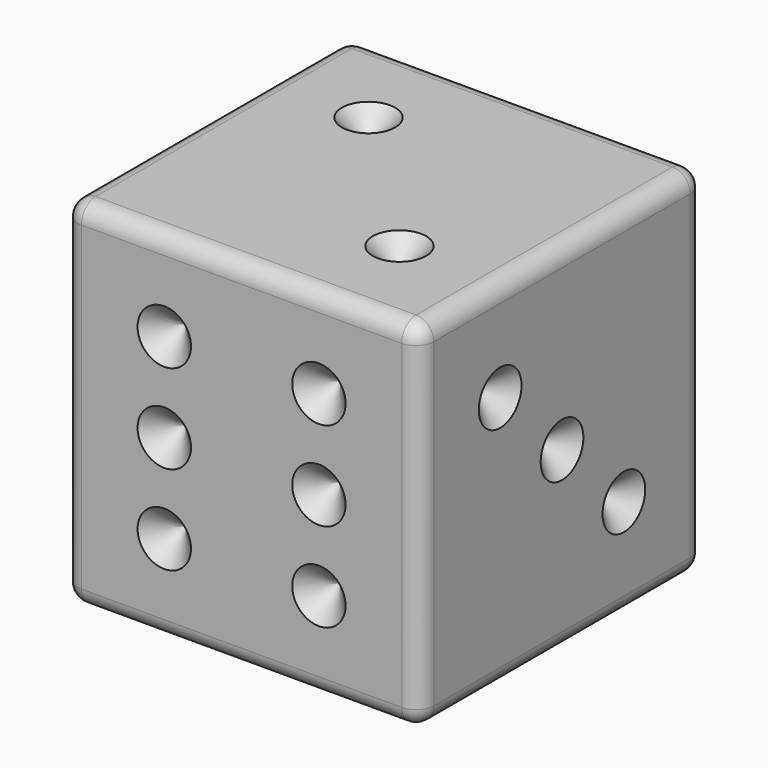
from build123d import *

# Parameters (mm, degrees)
F0_W      = 20
F0_H      = 20
F1_DEPTH  = 20
F2_R      = 1.5
F3_DEPTH  = 1.5
F4_R      = 1
F5_SIZE   = 1.49999
F6_R      = 1.5
F7_DEPTH  = 1.5
F8_SIZE   = 1.49999
F9_R      = 1.5
F10_DEPTH = 1.5
F11_SIZE  = 1.49999
F12_R     = 1.5
F13_DEPTH = 1.5
F14_SIZE  = 1.49999
F15_R     = 1.5
F16_DEPTH = 1.5
F17_SIZE  = 1.49999
F18_R     = 1.5
F19_DEPTH = 1.5
F20_SIZE  = 1.49999


# Not quite as in the source:
# - a fillet or chamfer is up to 0.001 mm smaller than in the source, because OpenCascade refuses the exact size


with BuildPart() as f1:
    # F0 (on Top) → F1 (new body)
    with BuildSketch(Plane.XY):
        with Locations((10, 10)):
            Rectangle(F0_W, F0_H)
    extrude(amount=F1_DEPTH)

    # F2 (on face) → F3 (cut)
    with BuildSketch(Plane.XY.offset(20)):
        with Locations((5.6568542495, 14.3431457505)):
            Circle(F2_R)
        with Locations((14.3431457505, 5.6568542495)):
            Circle(F2_R)
    extrude(amount=-F3_DEPTH, mode=Mode.SUBTRACT)

    # F4
    f4_edges = [f1.edges().sort_by_distance(p)[0] for p in [
        (10, 0, 20),
        (20, 0, 10),
        (0, 0, 10),
        (0, 10, 0),
        (0, 10, 20),
        (10, 20, 20),
        (20, 20, 10),
        (20, 10, 20),
        (10, 20, 0),
        (20, 10, 0),
        (0, 20, 10),
        (10, 0, 0),
    ]]
    fillet(f4_edges, radius=F4_R)

    # F5 (size 1.5 in the source; OpenCascade refuses exactly that, so slightly less here)
    f5_edges = [f1.edges().sort_by_distance(p)[0] for p in [
        (12.843146, 5.656854, 18.5),
        (4.156854, 14.343146, 18.5),
    ]]
    chamfer(f5_edges, length=F5_SIZE)

    # F6 (on face) → F7 (cut)
    with BuildSketch(Plane(origin=(0, 0, 0), x_dir=(1, 0, 0), z_dir=(0, 0, -1))):
        with Locations((5.6568542495, -5.6568542495)):
            Circle(F6_R)
        with Locations((14.3431457505, -5.6568542495)):
            Circle(F6_R)
        with Locations((14.3431457505, -14.3431457505)):
            Circle(F6_R)
        with Locations((5.6568542495, -14.3431457505)):
            Circle(F6_R)
        with Locations((10, -10)):
            Circle(F6_R)
    extrude(amount=-F7_DEPTH, mode=Mode.SUBTRACT)

    # F8 (size 1.5 in the source; OpenCascade refuses exactly that, so slightly less here)
    f8_edges = [f1.edges().sort_by_distance(p)[0] for p in [
        (4.156854, 5.656854, 1.5),
        (12.843146, 5.656854, 1.5),
        (8.5, 10, 1.5),
        (12.843146, 14.343146, 1.5),
        (4.156854, 14.343146, 1.5),
    ]]
    chamfer(f8_edges, length=F8_SIZE)

    # F9 (on face) → F10 (cut)
    with BuildSketch(Plane.YZ.offset(20)):
        with Locations((5.6568542495, 14.3431457505)):
            Circle(F9_R)
        with Locations((14.3431457505, 5.6568542495)):
            Circle(F9_R)
        with Locations((10, 10)):
            Circle(F9_R)
    extrude(amount=-F10_DEPTH, mode=Mode.SUBTRACT)

    # F11 (size 1.5 in the source; OpenCascade refuses exactly that, so slightly less here)
    f11_edges = [f1.edges().sort_by_distance(p)[0] for p in [
        (18.5, 4.156854, 14.343146),
        (18.5, 8.5, 10),
        (18.5, 12.843146, 5.656854),
    ]]
    chamfer(f11_edges, length=F11_SIZE)

    # F12 (on face) → F13 (cut)
    with BuildSketch(Plane(origin=(0, 20, 0), x_dir=(-1, 0, 0), z_dir=(0, 1, 0))):
        with Locations((-10, 10)):
            Circle(F12_R)
    extrude(amount=-F13_DEPTH, mode=Mode.SUBTRACT)

    # F14 (size 1.5 in the source; OpenCascade refuses exactly that, so slightly less here)
    f14_edges = [f1.edges().sort_by_distance(p)[0] for p in [
        (11.5, 18.5, 10),
    ]]
    chamfer(f14_edges, length=F14_SIZE)

    # F15 (on face) → F16 (cut)
    with BuildSketch(Plane(origin=(0, 0, 0), x_dir=(0, -1, 0), z_dir=(-1, 0, 0))):
        with Locations((-14.3431457505, 14.3431457505)):
            Circle(F15_R)
        with Locations((-5.6568542495, 14.3431457505)):
            Circle(F15_R)
        with Locations((-5.6568542495, 5.6568542495)):
            Circle(F15_R)
        with Locations((-14.3431457505, 5.6568542495)):
            Circle(F15_R)
    extrude(amount=-F16_DEPTH, mode=Mode.SUBTRACT)

    # F17 (size 1.5 in the source; OpenCascade refuses exactly that, so slightly less here)
    f17_edges = [f1.edges().sort_by_distance(p)[0] for p in [
        (1.5, 15.843146, 14.343146),
        (1.5, 7.156854, 14.343146),
        (1.5, 7.156854, 5.656854),
        (1.5, 15.843146, 5.656854),
    ]]
    chamfer(f17_edges, length=F17_SIZE)

    # F18 (on face) → F19 (cut)
    with BuildSketch(Plane.XZ):
        with Locations((5.6568542495, 10)):
            Circle(F18_R)
        with Locations((5.6568542495, 5)):
            Circle(F18_R)
        with Locations((14.3431457505, 10)):
            Circle(F18_R)
        with Locations((14.3431457505, 5)):
            Circle(F18_R)
        with Locations((5.6568542495, 15)):
            Circle(F18_R)
        with Locations((14.3431457505, 15)):
            Circle(F18_R)
    extrude(amount=-F19_DEPTH, mode=Mode.SUBTRACT)

    # F20 (size 1.5 in the source; OpenCascade refuses exactly that, so slightly less here)
    f20_edges = [f1.edges().sort_by_distance(p)[0] for p in [
        (4.156854, 1.5, 15),
        (12.843146, 1.5, 15),
        (12.843146, 1.5, 10),
        (4.156854, 1.5, 10),
        (12.843146, 1.5, 5),
        (4.156854, 1.5, 5),
    ]]
    chamfer(f20_edges, length=F20_SIZE)


solid = f1.part
